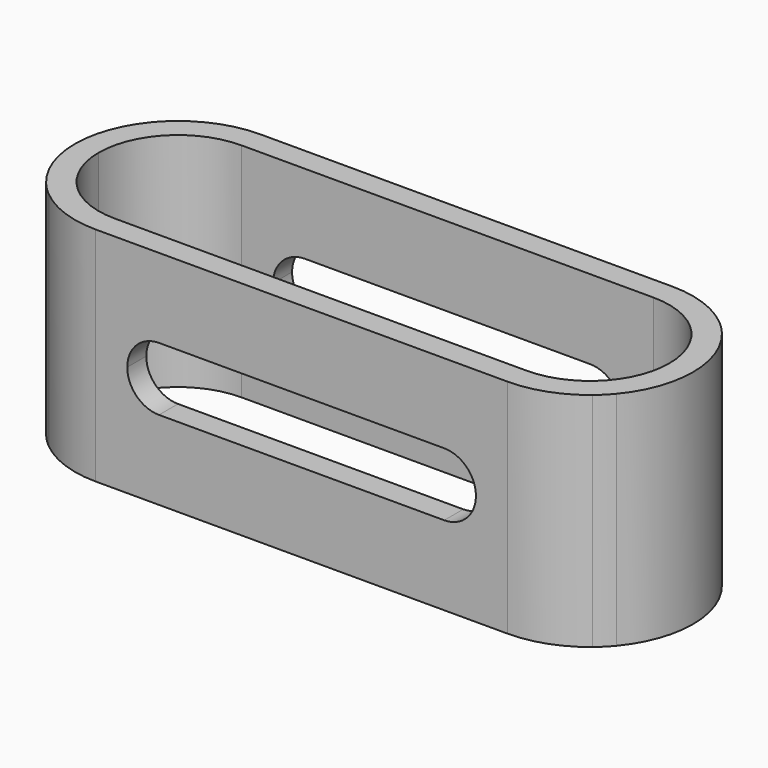
from build123d import *

# Parameters (mm, degrees)
F1_DEPTH = 7
F2_W     = 11
F2_H     = 2
F3_DEPTH = 6.501
F4_R     = 0.99999


# Not quite as in the source:
# - a fillet or chamfer is up to 0.001 mm smaller than in the source, because OpenCascade refuses the exact size


with BuildPart() as f1:
    # F0 (on Top) → F1 (new body)
    with BuildSketch(Plane.XY):
        with BuildLine():
            Line((-2.0766559657, 0), (0, 0))
            Line((0, 0), (13, 0))
            Line((13, 0), (15.0766559657, 0))
            ThreePointArc((15.0766559657, 0), (14.1039701083, 0.5567548152), (13, 0.75))
            Line((13, 0.75), (0, 0.75))
            ThreePointArc((0, 0.75), (-1.1039701083, 0.5567548152), (-2.0766559657, 0))
        make_face()
        with BuildLine():
            ThreePointArc((-2.5, -2.5), (-1.767766953, -0.732233047), (0, 0))
            Line((0, 0), (-2.0766559657, 0))
            ThreePointArc((-2.0766559657, 0), (-2.2980970389, -0.2019029611), (-2.5, -0.4233440343))
            Line((-2.5, -0.4233440343), (-2.5, -2.5))
        make_face()
        with BuildLine():
            ThreePointArc((0, -5), (-1.767766953, -4.267766953), (-2.5, -2.5))
            Line((-2.5, -2.5), (-2.5, -4.5766559657))
            ThreePointArc((-2.5, -4.5766559657), (-2.2980970389, -4.7980970389), (-2.0766559657, -5))
            Line((-2.0766559657, -5), (0, -5))
        make_face()
        with BuildLine():
            Line((-2.5, -4.5766559657), (-2.5, -2.5))
            Line((-2.5, -2.5), (-2.5, -0.4233440343))
            ThreePointArc((-2.5, -0.4233440343), (-3.25, -2.5), (-2.5, -4.5766559657))
        make_face()
        with BuildLine():
            Line((15.5, -0.4233440343), (15.5, -2.5))
            Line((15.5, -2.5), (15.5, -4.5766559657))
            ThreePointArc((15.5, -4.5766559657), (16.25, -2.5), (15.5, -0.4233440343))
        make_face()
        with BuildLine():
            Line((15.0766559657, 0), (13, 0))
            ThreePointArc((13, 0), (14.767766953, -0.732233047), (15.5, -2.5))
            Line((15.5, -2.5), (15.5, -0.4233440343))
            ThreePointArc((15.5, -0.4233440343), (15.2980970389, -0.2019029611), (15.0766559657, 0))
        make_face()
        with BuildLine():
            Line((15.5, -4.5766559657), (15.5, -2.5))
            ThreePointArc((15.5, -2.5), (14.767766953, -4.267766953), (13, -5))
            Line((13, -5), (15.0766559657, -5))
            ThreePointArc((15.0766559657, -5), (15.2980970389, -4.7980970389), (15.5, -4.5766559657))
        make_face()
        with BuildLine():
            Line((13, -5), (0, -5))
            Line((0, -5), (-2.0766559657, -5))
            ThreePointArc((-2.0766559657, -5), (-1.1039701083, -5.5567548152), (0, -5.75))
            Line((0, -5.75), (13, -5.75))
            ThreePointArc((13, -5.75), (14.1039701083, -5.5567548152), (15.0766559657, -5))
            Line((15.0766559657, -5), (13, -5))
        make_face()
    extrude(amount=F1_DEPTH)

    # F2 (on face) → F3 (cut, through all)
    with BuildSketch(Plane.XZ.offset(5.75)):
        with Locations((6.5, 3.5)):
            Rectangle(F2_W, F2_H)
    extrude(amount=-F3_DEPTH, mode=Mode.SUBTRACT)

    # F4 (radius 1 in the source; OpenCascade refuses exactly that, so slightly less here)
    f4_edges = [f1.edges().sort_by_distance(p)[0] for p in [
        (1, -5.375, 4.5),
        (1, -5.375, 2.5),
        (12, -5.375, 2.5),
        (12, 0.375, 4.5),
        (12, -5.375, 4.5),
        (12, 0.375, 2.5),
        (1, 0.375, 2.5),
        (1, 0.375, 4.5),
    ]]
    fillet(f4_edges, radius=F4_R)


solid = f1.part
